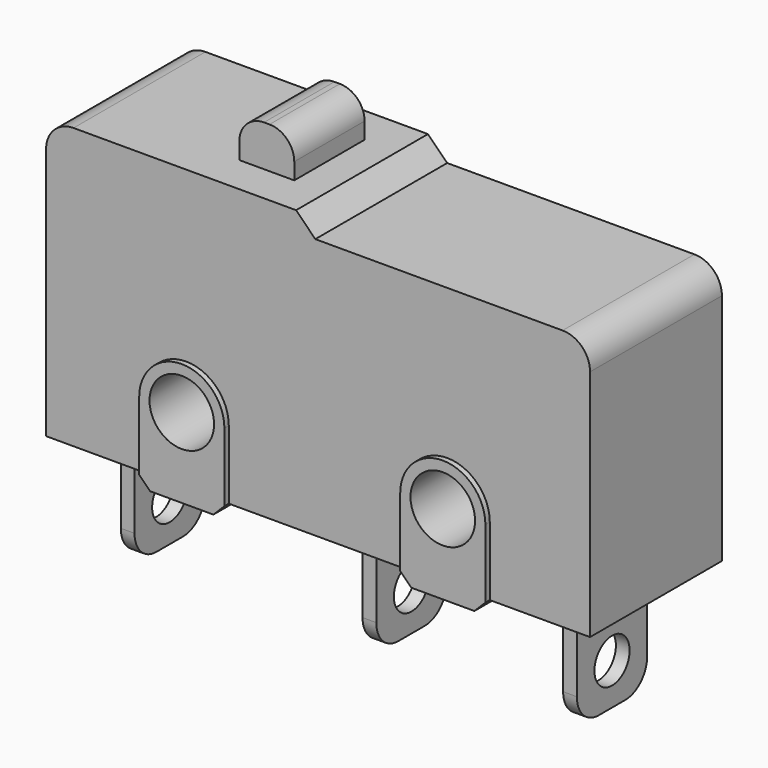
from build123d import *

# Parameters (mm, degrees)
F0_W      = 19.8
F0_H      = 10.2
F1_DEPTH  = 6
F3_DEPTH  = 0.2
F5_DEPTH  = 6.4
F6_DEPTH  = 6.4
F7_SIZE   = 0.39999
F9_DEPTH  = 6.201
F10_R     = 1
F12_D     = 2.35
F14_D     = 2.35
F15_W     = 2
F15_H     = 3.2
F16_DEPTH = 1.5
F17_R     = 0.9
F18_W     = 0.5
F18_H     = 3.2
F19_DEPTH = 4
F21_D     = 1.6
F22_R     = 1


# Not quite as in the source:
# - a fillet or chamfer is up to 0.001 mm smaller than in the source, because OpenCascade refuses the exact size


with BuildPart() as f1:
    # F0 (on Front) → F1 (new body)
    with BuildSketch(Plane.XZ):
        with Locations((9.9, 5.1)):
            Rectangle(F0_W, F0_H)
    extrude(amount=F1_DEPTH)

    # F2 (on face) → F3 (join)
    with BuildSketch(Plane.XZ.offset(6)):
        with BuildLine():
            ThreePointArc((3.55, 2.5), (5.1, 0.95), (6.65, 2.5))
            ThreePointArc((6.65, 2.5), (5.1, 4.05), (3.55, 2.5))
        make_face()
        with BuildLine():
            Line((6.65, -0.4), (6.65, 2.5))
            ThreePointArc((6.65, 2.5), (5.1, 0.95), (3.55, 2.5))
            Line((3.55, 2.5), (3.55, -0.4))
            Line((3.55, -0.4), (6.65, -0.4))
        make_face()
        with BuildLine():
            ThreePointArc((13.05, 2.5), (14.6, 0.95), (16.15, 2.5))
            ThreePointArc((16.15, 2.5), (14.6, 4.05), (13.05, 2.5))
        make_face()
        with BuildLine():
            Line((16.15, -0.4), (16.15, 2.5))
            ThreePointArc((16.15, 2.5), (14.6, 0.95), (13.05, 2.5))
            Line((13.05, 2.5), (13.05, -0.4))
            Line((13.05, -0.4), (16.15, -0.4))
        make_face()
    extrude(amount=F3_DEPTH)

    # F4 (on face) → F5 (join)
    with BuildSketch(Plane.XZ.offset(6.2)):
        with BuildLine():
            Line((6.65, -0.4), (6.65, 2.5))
            ThreePointArc((6.65, 2.5), (5.1, 4.05), (3.55, 2.5))
            Line((3.55, 2.5), (3.55, -0.4))
            Line((3.55, -0.4), (6.65, -0.4))
        make_face()
    extrude(amount=-F5_DEPTH)

    # F6 (add): a face of the model
    f6_faces = [f1.faces().sort_by_distance(p)[0] for p in [
        (14.6, -6.2, 1.6732176073),
    ]]
    extrude(f6_faces, amount=-F6_DEPTH)

    # F7 (size 0.4 in the source; OpenCascade refuses exactly that, so slightly less here)
    f7_edges = [f1.edges().sort_by_distance(p)[0] for p in [
        (3.55, -3, -0.4),
        (6.65, -3, -0.4),
        (13.05, -3, -0.4),
        (16.15, -3, -0.4),
    ]]
    chamfer(f7_edges, length=F7_SIZE)

    # F8 (on face) → F9 (cut, through all)
    with BuildSketch(Plane.XZ.offset(6)):
        Polygon((19.8, 10.2), (9.1, 10.2), (9.8, 9.5), (19.8, 9.5), align=None)
    extrude(amount=-F9_DEPTH, mode=Mode.SUBTRACT)

    # F10
    f10_edges = [f1.edges().sort_by_distance(p)[0] for p in [
        (0, -3, 10.2),
        (19.8, -3, 9.5),
    ]]
    fillet(f10_edges, radius=F10_R)

    # F12 (through all)
    with Locations(Plane.XZ.offset(6.2)):
        with Locations((5.1, 2.5)):
            Hole(F12_D / 2)

    # F14 (through all)
    with Locations(Plane.XZ.offset(6.2)):
        with Locations((14.6, 2.5)):
            Hole(F14_D / 2)

    # F15 (on face) → F16 (join)
    with BuildSketch(Plane.XY.offset(10.2)):
        with Locations((6.9132626522, -3)):
            Rectangle(F15_W, F15_H)
    extrude(amount=F16_DEPTH)

    # F17
    f17_edges = [f1.edges().sort_by_distance(p)[0] for p in [
        (5.913263, -3, 11.7),
        (7.913263, -3, 11.7),
    ]]
    fillet(f17_edges, radius=F17_R)

    # F18 (on face) → F19 (join)
    with BuildSketch(Plane(origin=(0, 0, 0), x_dir=(1, 0, 0), z_dir=(0, 0, -1))):
        with Locations((1.85, 3)):
            Rectangle(F18_W, F18_H)
        with Locations((10.65, 3)):
            Rectangle(F18_W, F18_H)
        with Locations((17.95, 3)):
            Rectangle(F18_W, F18_H)
    extrude(amount=F19_DEPTH)

    # F21 (through all)
    with Locations(Plane(origin=(1.6, 0, 0), x_dir=(0, -1, 0), z_dir=(-1, 0, 0))):
        with Locations((3, -2.4945095647)):
            Hole(F21_D / 2)

    # F22
    f22_edges = [f1.edges().sort_by_distance(p)[0] for p in [
        (17.95, -4.6, -4),
        (10.65, -4.6, -4),
        (1.85, -4.6, -4),
        (1.85, -1.4, -4),
        (10.65, -1.4, -4),
        (17.95, -1.4, -4),
    ]]
    fillet(f22_edges, radius=F22_R)


solid = f1.part
